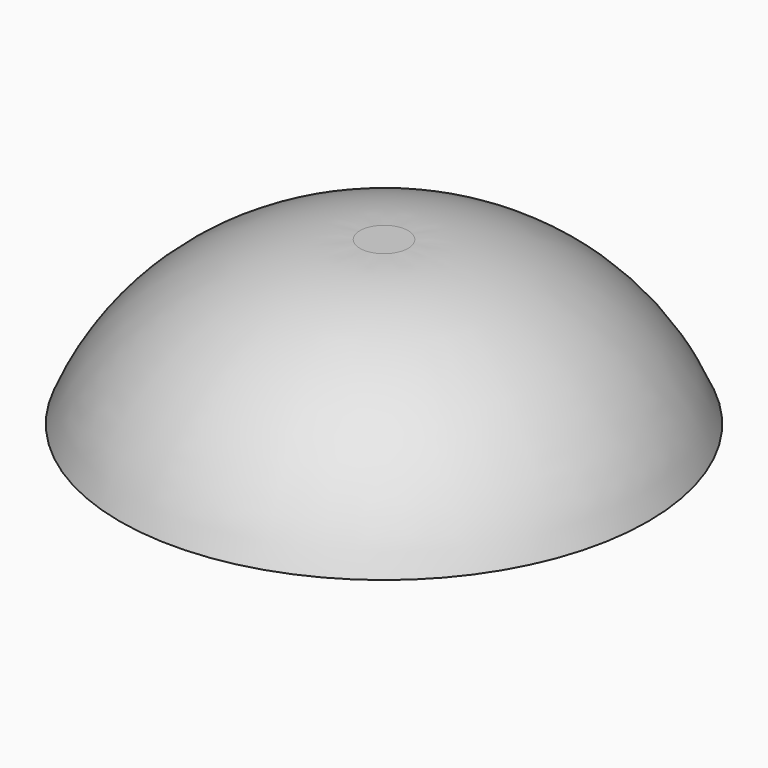
from build123d import *

# Parameters (mm, degrees)
F0_R     = 48.8103763307
F1_DEPTH = 30
F3_T     = -1


# Not quite as in the source:
# - a fillet or chamfer that OpenCascade refuses, or shapes differently, is made with other operations: its cross-section is extruded or revolved along the edge and cut away or added


with BuildPart() as f1:
    # F0 (on Top) → F1 (new body)
    with BuildSketch(Plane.XY):
        Circle(F0_R)
    extrude(amount=F1_DEPTH)

    # F2: fillet of radius 47.801428535 on 1 edges, made by hand

    # F2_s1 → F2_t2 (revolve, cut)
    with BuildSketch(Plane.XZ):
        with BuildLine():
            ThreePointArc((48.8103763307, 0), (31.2245200627, 21.7959847891), (4.4472642656, 30))
            Line((4.4472642656, 30), (4.4472642656, 30.9560285707))
            Line((4.4472642656, 30.9560285707), (48.8103763307, 30.9560285707))
            Line((48.8103763307, 30.9560285707), (49.7664049014, 30))
            ThreePointArc((49.7664049014, 30), (49.7664049014, 15), (49.697638572, 0.3560285707))
            Line((49.697638572, 0.3560285707), (48.8103763307, 0))
        make_face()
    revolve(axis=Axis((0, 0, 30), (0, 0, 1)), mode=Mode.SUBTRACT)

    # F3
    f3_openings = [f1.faces().sort_by_distance(p)[0] for p in [
        (0, 0, 0),
    ]]
    offset(amount=F3_T, openings=f3_openings)


solid = f1.part
